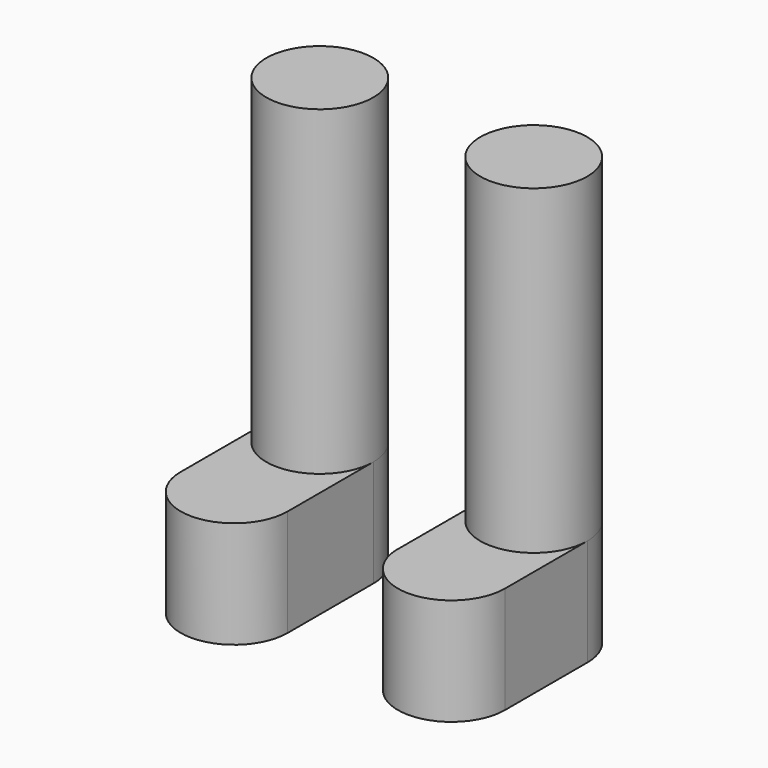
from build123d import *
from build123d import SkipClean  # not in build123d's __all__

# Parameters (mm, degrees)
F0_R     = 5
F1_DEPTH = 30
F3_DEPTH = 10
F5_DEPTH = 10


with BuildPart() as f1:
    # F0 (on Top) → F1 (new body)
    with BuildSketch(Plane.XY):
        with Locations((10.087849088, 0)):
            Circle(F0_R)
    extrude(amount=-F1_DEPTH)

    # F4 (on face) → F5 (join)
    with BuildSketch(Plane(origin=(0, 0, -30), x_dir=(1, 0, 0), z_dir=(0, 0, -1))):
        with BuildLine():
            Line((5.087849088, 10), (5.087849088, 0))
            ThreePointArc((5.087849088, 0), (10.087849088, -5), (15.087849088, 0))
            Line((15.087849088, 0), (15.087849088, 9.61173255))
            ThreePointArc((15.087849088, 9.61173255), (10.2745915071, 14.615499921), (5.087849088, 10))
        make_face()
    with SkipClean():  # cleaning this boolean's faces spoils the solid; the shape is the same uncleaned
        extrude(amount=F5_DEPTH)


with BuildPart() as f1b:
    # F0 (on Top) → F1, piece 2 (new body)
    with BuildSketch(Plane.XY):
        with Locations((-9.912150912, 0)):
            Circle(F0_R)
    extrude(amount=-F1_DEPTH)

    # F2 (on face) → F3 (join)
    with BuildSketch(Plane(origin=(0, 0, -30), x_dir=(1, 0, 0), z_dir=(0, 0, -1))):
        with BuildLine():
            Line((-14.912150912, 10), (-14.912150912, 0))
            ThreePointArc((-14.912150912, 0), (-9.912150912, -5), (-4.912150912, 0))
            Line((-4.912150912, 0), (-4.912150912, 10))
            ThreePointArc((-4.912150912, 10), (-9.912150912, 15), (-14.912150912, 10))
        make_face()
    with SkipClean():  # cleaning this boolean's faces spoils the solid; the shape is the same uncleaned
        extrude(amount=F3_DEPTH)


solid = Compound([f1.part, f1b.part])
